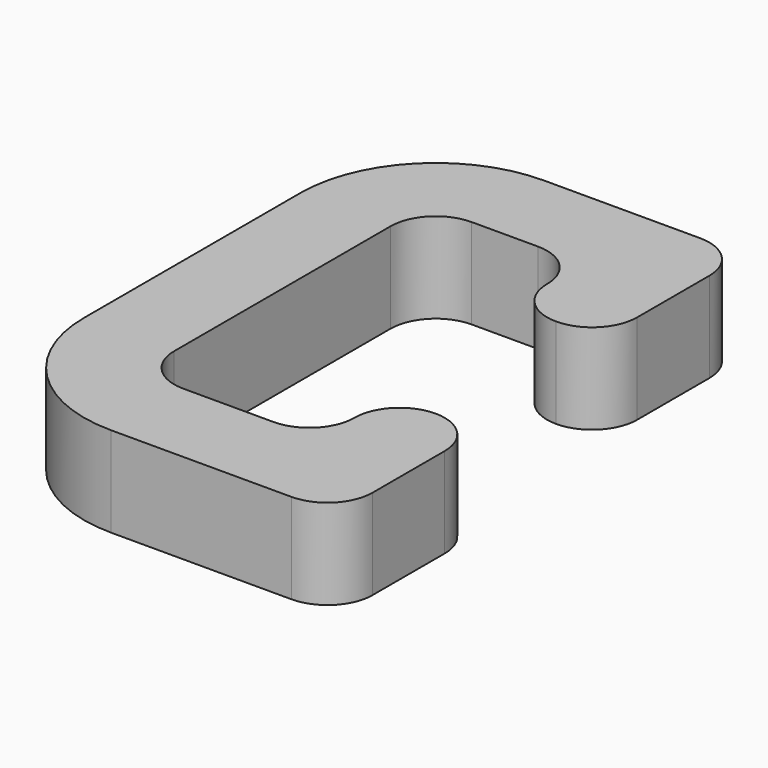
from build123d import *

# Parameters (mm, degrees)
F0_W     = 10
F0_H     = 10
F1_DEPTH = 10
F2_R     = 4.99999
F3_R     = 5
F4_R     = 5
F5_R     = 15


# Not quite as in the source:
# - a fillet or chamfer is up to 0.001 mm smaller than in the source, because OpenCascade refuses the exact size


with BuildPart() as f1:
    # F0 (on Top) → F1 (new body)
    with BuildSketch(Plane.XY):
        Polygon((10.8962109051, 41.5868479488), (10.8962109051, 31.5868479488), (10.8962109051, 21.5868479488), (20.8962109051, 21.5868479488), (20.8962109051, 41.5868479488), align=None)
        Polygon((-16.4567323537, 41.5868479488), (-16.4567323537, 31.5868479488), (-6.4567323537, 31.5868479488), (10.8962109051, 31.5868479488), (10.8962109051, 41.5868479488), align=None)
        Polygon((-6.4567323537, 31.5868479488), (-16.4567323537, 31.5868479488), (-16.4567323537, -18.4131520512), (-6.4567323537, -18.4131520512), (-6.4567323537, -8.4131520512), align=None)
        Polygon((13.5432676463, -8.4131520512), (-6.4567323537, -8.4131520512), (-6.4567323537, -18.4131520512), (23.5432676463, -18.4131520512), (23.5432676463, -8.4131520512), align=None)
        with Locations((18.5432676463, -3.4131520512)):
            Rectangle(F0_W, F0_H)
    extrude(amount=F1_DEPTH)

    # F2 (radius 5 in the source; OpenCascade refuses exactly that, so slightly less here)
    f2_edges = [f1.edges().sort_by_distance(p)[0] for p in [
        (13.543268, 1.586848, 5),
        (10.896211, 21.586848, 5),
        (10.896211, 31.586848, 5),
        (-6.456732, 31.586848, 5),
        (-6.456732, -8.413152, 5),
        (13.543268, -8.413152, 5),
    ]]
    fillet(f2_edges, radius=F2_R)

    # F3
    f3_edges = [f1.edges().sort_by_distance(p)[0] for p in [
        (23.543268, 1.586848, 5),
        (20.896211, 21.586848, 5),
    ]]
    fillet(f3_edges, radius=F3_R)

    # F4
    f4_edges = [f1.edges().sort_by_distance(p)[0] for p in [
        (23.543268, -18.413152, 5),
        (20.896211, 41.586848, 5),
    ]]
    fillet(f4_edges, radius=F4_R)

    # F5
    f5_edges = [f1.edges().sort_by_distance(p)[0] for p in [
        (-16.456732, -18.413152, 5),
        (-16.456732, 41.586848, 5),
    ]]
    fillet(f5_edges, radius=F5_R)


solid = f1.part
